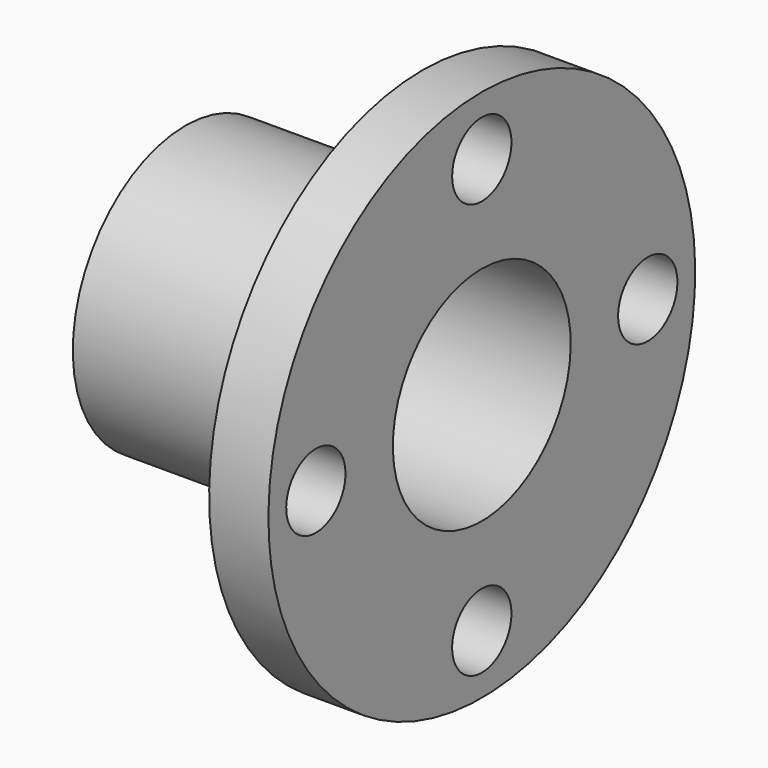
from build123d import *

# Parameters (mm, degrees)
F2_R            = 12.5
F3_DEPTH        = 85
F3_COPIES_COUNT = 4


# Not quite as in the source:
# - a pattern or mirror of a feature is missing from the dataset's text; its kind, count and spacing are read off the source's solid


with BuildPart() as f1:
    # F0 (on Front) → F1 (revolve)
    with BuildSketch(Plane.XZ):
        Polygon((-100, 47.5), (-100, 37.5), (0, 37.5), (0, 90), (-20, 90), (-20, 47.5), align=None)
    revolve(axis=Axis((-54.4903725386, 0, 0), (-1, 0, 0)))

    # F2 (on face) → F3 (cut)
    with BuildSketch(Plane(origin=(-20, 0, 0), x_dir=(0, -1, 0), z_dir=(-1, 0, 0))):
        with Locations((0, 70)):
            Circle(F2_R)
    f3 = extrude(amount=-F3_DEPTH, mode=Mode.SUBTRACT)

    # F3_copies: F3 ×4 about axis
    f3_copies_axis = Axis((0, 0, 0), (1, 0, 0))
    for i in range(1, F3_COPIES_COUNT):
        add(f3.rotate(f3_copies_axis, i * 360 / F3_COPIES_COUNT), mode=Mode.SUBTRACT)


solid = f1.part
